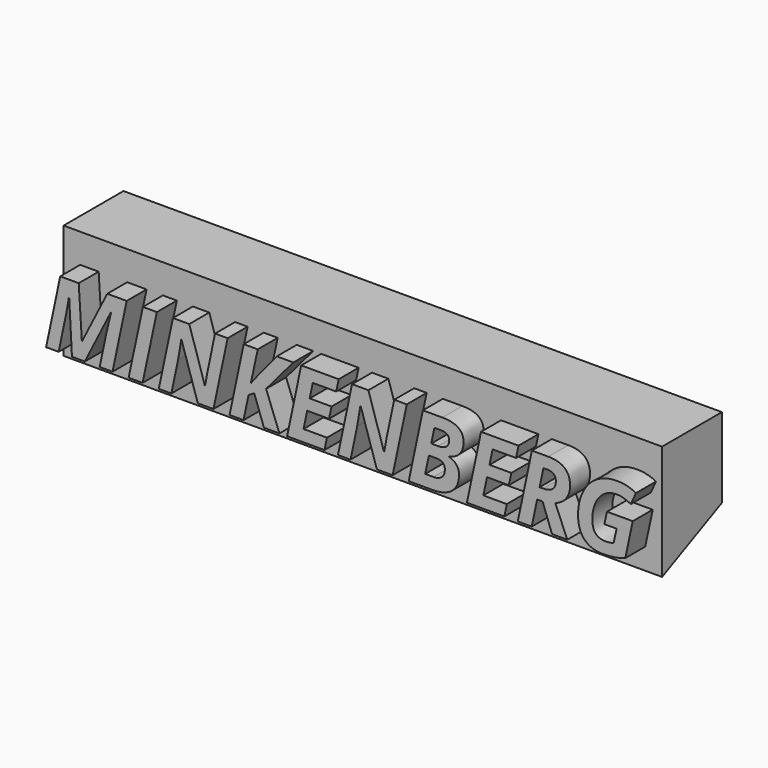
from build123d import *

# Parameters (mm, degrees)
F0_W         = 120
F0_H         = 30
F1_DEPTH     = 15
F2_TEXT_SIZE = 18.8078561983
F3_DEPTH     = 5
F4_T1_DEPTH  = 275.4585282854


# Not quite as in the source:
# - a fillet or chamfer that OpenCascade refuses, or shapes differently, is made with other operations: its cross-section is extruded or revolved along the edge and cut away or added
# - Text() gives the source's letters only with a copy of the font that has no kerning and outlines rounded to 1/6400 em; it was checked with that copy


with BuildPart() as f1:
    # F0 (on Front) → F1 (new body)
    with BuildSketch(Plane.XZ):
        with Locations((-0.1326536376, 15)):
            Rectangle(F0_W, F0_H)
    extrude(amount=F1_DEPTH)

    # F2 (on face) → F3 (join)
    with BuildSketch(Plane.XZ.offset(15)):
        with Locations((-60.1326536376, 10.7203700548)):
            Text('MINKENBERG', F2_TEXT_SIZE, font='Open Sans', font_style=FontStyle.BOLDITALIC, text_align=(TextAlign.LEFT, TextAlign.BOTTOM))
    extrude(amount=F3_DEPTH)

    # F4: chamfer of 30 x 13.9892297446 on 1 edges, made by hand

    # F4_s2 → F4_t1 (cut)
    with BuildSketch(Plane.YZ.offset(-137.8619177803)):
        Polygon((0, 13.9892297446), (-30, 0), (0, 0), align=None)
    extrude(amount=F4_T1_DEPTH, mode=Mode.SUBTRACT)


solid = f1.part
